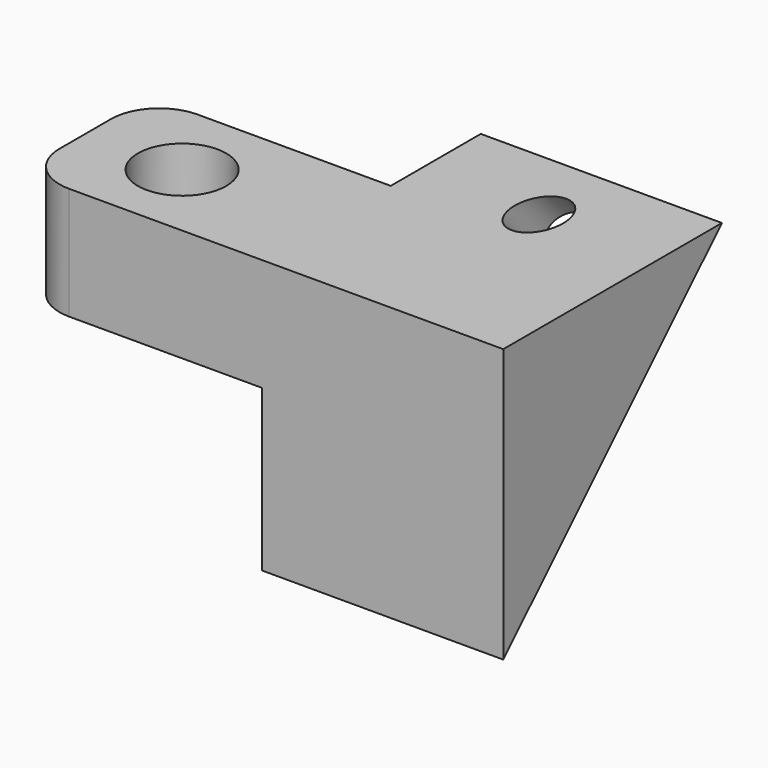
from build123d import *

# Parameters (mm, degrees)
F0_W     = 30
F0_H     = 10
F0_R     = 2.75
F1_DEPTH = 7
F3_DEPTH = 15
F4_R     = 3
F5_R     = 1.5
F6_DEPTH = 25


# Not quite as in the source:
# - a feature names something its author has since deleted; it is built from what else it names


with BuildPart() as f1:
    # F0 (on Top) → F1 (new body)
    with BuildSketch(Plane.XY):
        with Locations((-23.3256115019, 35.3867347538)):
            Rectangle(F0_W, F0_H)
        with Locations((-32.3030129075, 35.3867347538)):
            Circle(F0_R, mode=Mode.SUBTRACT)
    extrude(amount=F1_DEPTH)

    # F2 (on face) → F3 (join)
    with BuildSketch(Plane.YZ.offset(-8.3256115019)):
        Polygon((30.3867347538, -10), (40.3867347538, 0), (30.3867347538, 0), align=None)
        Polygon((40.3867347538, 7), (40.3867347538, 0), (47.3867347538, 7), align=None)
    extrude(amount=-F3_DEPTH)

    # F4
    f4_edges = [f1.edges().sort_by_distance(p)[0] for p in [
        (-38.325612, 40.386735, 3.5),
        (-38.325612, 30.386735, 3.5),
    ]]
    fillet(f4_edges, radius=F4_R)

    # F5 (on face) → F6 (cut)
    with BuildSketch(Plane(origin=(0, 20.1933673769, -20.1933673769), x_dir=(1, 0, 0), z_dir=(0, 0.7071067812, -0.7071067812))):
        with Locations((-15.8256115019, -35.0243411958)):
            Circle(F5_R)
    extrude(amount=-F6_DEPTH, mode=Mode.SUBTRACT)


solid = f1.part
